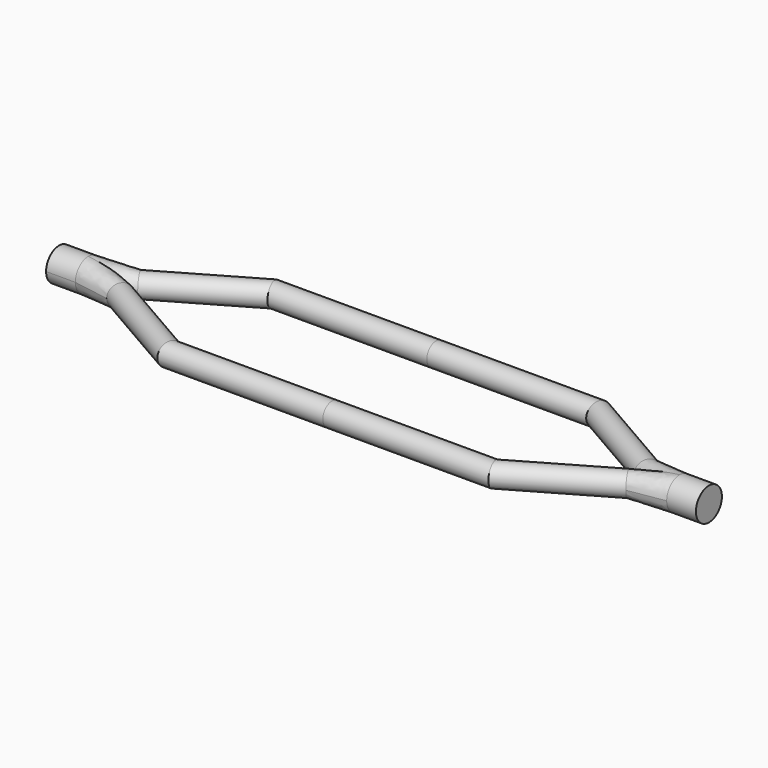
from build123d import *

# Parameters (mm, degrees)
F1_R      = 0.5
F8_R      = 0.35355
F2_FACE_R = 0.5
F9_FACE_R = 0.35355


# Not quite as in the source:
# - a feature names something its author has since deleted; it is built from what else it names


with BuildPart() as f2:
    # F2: sweep along a path in F0
    with BuildLine(Plane.XY) as f2_path:
        Line((0, 3.5), (0.9, 3.5))
    # F1 (on Right) → F2 (sweep)
    with BuildSketch(Plane.YZ):
        with Locations((3.5, 0)):
            Circle(F1_R)
    sweep(path=f2_path.line)



with BuildPart() as f9:
    # F9: sweep along a path in F0
    with BuildLine(Plane.XY) as f9_path:
        Line((2.1874061588, 3.8761481887), (5, 5.5))
        Line((5, 5.5), (10, 5.5))
    # F8 (on face) → F9 (sweep)
    with BuildSketch(Plane(origin=(3.3189760192, 1.9162116981, 0), x_dir=(-0.5, 0.8660254038, 0), z_dir=(0.8660254038, 0.5, 0))):
        with Locations((2.2631397208, 0)):
            Circle(F8_R)
    sweep(path=f9_path.line, transition=Transition.RIGHT)


with BuildPart() as f2_1:
    add(f2.part)

    add(f9.part)  # F10 merges F9
    # F2_face (on face) → F10 section 0
    with BuildSketch(Plane(origin=(0.9, 3.5, 0), x_dir=(0, 1, 0), z_dir=(1, 0, 0))):
        Circle(F2_FACE_R)
    # F9_face (on face) → F10 section 1
    with BuildSketch(Plane(origin=(2.1874061588, 3.8761481887, 0), x_dir=(0.5, -0.8660254038, 0), z_dir=(-0.8660254038, -0.5, 0))):
        Circle(F9_FACE_R)
    loft()

    # F11: F2 across plane


with BuildPart() as f2_2:
    add(f2_1.part)
    add(f2_1.part.mirror(Plane.YZ.offset(10)))

    # F12: F2 across plane


with BuildPart() as f2_3:
    add(f2_2.part)
    add(f2_2.part.mirror(Plane.XZ.offset(-3.5)))


solid = f2_3.part
